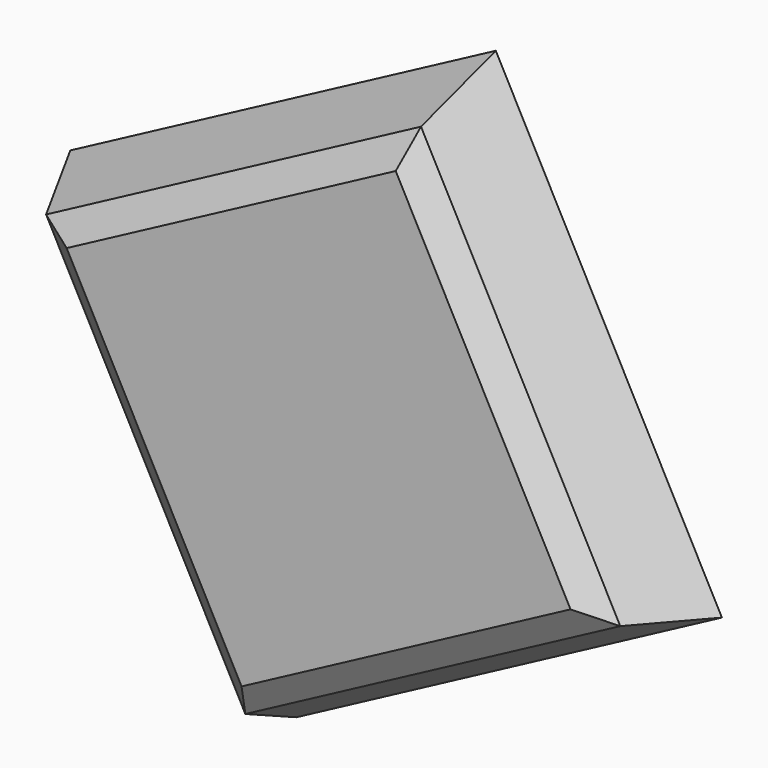
from build123d import *

# Parameters (mm, degrees)
F1_DEPTH = 25.4
F1_TAPER = -20
F2_SIZE  = 5.08


# Not quite as in the source:
# - a feature names something its author has since deleted; it is built from what else it names


with BuildPart() as f1:
    # F0 (on Front) → F1 (new body)
    with BuildSketch(Plane.XZ):
        Polygon((-22.3139226437, -8.2820653915), (72.9333236814, 42.3373356462), (22.3139226437, 137.5845819712), (-72.9333236814, 86.9651809335), align=None)
    extrude(amount=-F1_DEPTH, taper=F1_TAPER)

    # F2
    f2_edges = [f1.edges().sort_by_distance(p)[0] for p in [
        (25.309701, 0, 17.027635),
        (47.623623, 0, 89.960959),
        (-25.309701, 0, 112.274881),
        (-47.623623, 0, 39.341558),
    ]]
    chamfer(f2_edges, length=F2_SIZE)


solid = f1.part
